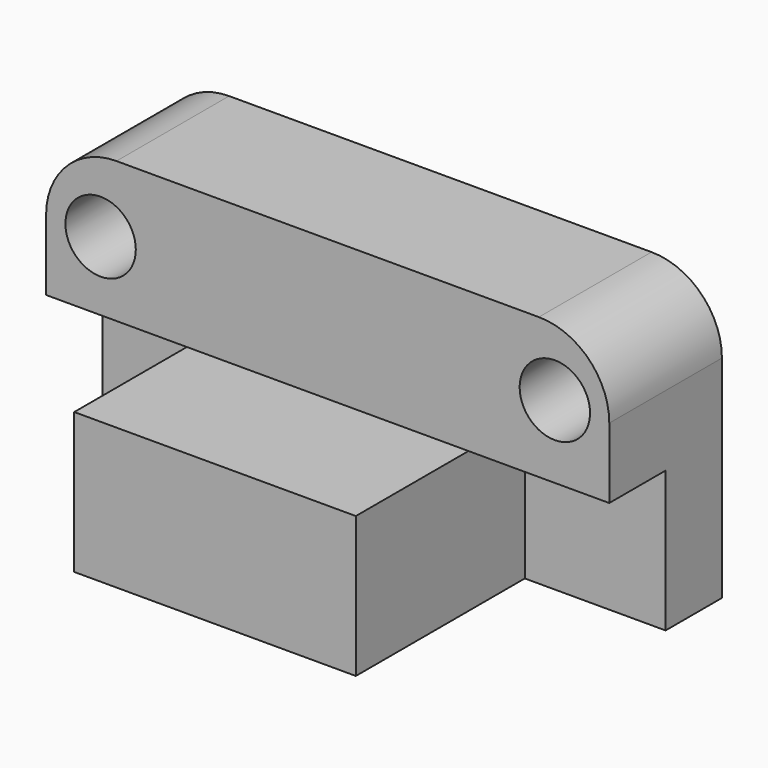
from build123d import *

# Parameters (mm, degrees)
F0_W      = 101.6
F0_H      = 101.6
F1_DEPTH  = 50.8
F2_W      = 25.4
F2_H      = 50.8
F3_DEPTH  = 50.8
F4_W      = 25.4
F4_H      = 50.8
F5_DEPTH  = 50.8
F7_DEPTH  = 25.4
F8_DEPTH  = 25.4
F10_DEPTH = 25.4
F11_R     = 12.7
F12_DEPTH = 50.8
F14_DEPTH = 50.8
F15_R     = 25.4
F16_R     = 25.4


with BuildPart() as f1:
    # F0 (on Top) → F1 (new body)
    with BuildSketch(Plane.XY):
        with Locations((-39.0884162307, 27.9844595671)):
            Rectangle(F0_W, F0_H)
    extrude(amount=F1_DEPTH)

    # F2 (on face) → F3 (join)
    with BuildSketch(Plane.YZ.offset(11.7115837693)):
        with Locations((66.0844595671, 25.4)):
            Rectangle(F2_W, F2_H)
    extrude(amount=F3_DEPTH)

    # F4 (on face) → F5 (join)
    with BuildSketch(Plane(origin=(-89.8884162307, 0, 0), x_dir=(0, -1, 0), z_dir=(-1, 0, 0))):
        with Locations((-66.0844595671, 25.4)):
            Rectangle(F4_W, F4_H)
    extrude(amount=F5_DEPTH)

    # F6 (on face) → F7 (join)
    with BuildSketch(Plane.XY.offset(50.8)):
        Polygon((-140.6884162307, 53.3844595671), (-89.8884162307, 53.3844595671), (11.7115837693, 53.3844595671), (62.5115837693, 53.3844595671), (62.5115837693, 78.7844595671), (-140.6884162307, 78.7844595671), align=None)
    extrude(amount=F7_DEPTH)

    # F8 (add): a face of the model
    f8_faces = [f1.faces().sort_by_distance(p)[0] for p in [
        (-39.0884162307, 66.0844595671, 76.2),
    ]]
    extrude(f8_faces, amount=F8_DEPTH)

    # F9 (on face) → F10 (join)
    with BuildSketch(Plane.XZ.offset(-53.3844595671)):
        Polygon((-140.6884162307, 50.8), (-89.8884162307, 50.8), (11.7115837693, 50.8), (62.5115837693, 50.8), (62.5115837693, 101.6), (-140.6884162307, 101.6), align=None)
    extrude(amount=F10_DEPTH)

    # F11 (on face) → F12 (cut)
    with BuildSketch(Plane.XZ.offset(-27.9844595671)):
        with Locations((-121.0152357817, 75.7217407227)):
            Circle(F11_R)
    extrude(amount=-F12_DEPTH, mode=Mode.SUBTRACT)

    # F13 (on face) → F14 (cut)
    with BuildSketch(Plane.XZ.offset(-27.9844595671)):
        with BuildLine():
            ThreePointArc((55.5737721028, 77.0839367255), (30.1813854063, 77.523618368), (55.5433280167, 76.2051005946))
            ThreePointArc((55.5433280167, 76.2051005946), (55.5661587993, 76.6442550829), (55.5737721028, 77.0839367255))
        make_face()
    extrude(amount=-F14_DEPTH, mode=Mode.SUBTRACT)

    # F15
    f15_edges = [f1.edges().sort_by_distance(p)[0] for p in [
        (62.511584, 53.38446, 101.6),
    ]]
    fillet(f15_edges, radius=F15_R)

    # F16
    f16_edges = [f1.edges().sort_by_distance(p)[0] for p in [
        (-140.688416, 53.38446, 101.6),
    ]]
    fillet(f16_edges, radius=F16_R)


solid = f1.part
